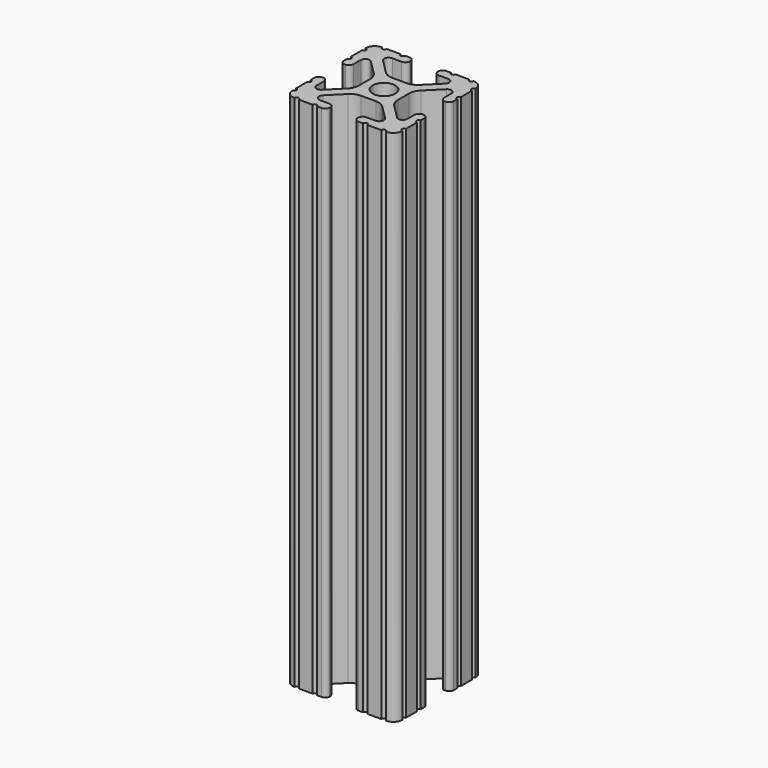
from build123d import *

# Parameters (mm, degrees)
F0_R     = 2.6035
F1_DEPTH = 120


# Not quite as in the source:
# - ends of sketch curves that miss each other by under 0.0002 mm in the source are joined


with BuildPart() as f1:
    # F0 (on Top) → F1 (new body)
    with BuildSketch(Plane.XY):
        with BuildLine():
            ThreePointArc((-3.9522606035, -5.4236922052), (-2.9229262099, -4.7369294977), (-1.7092422, -4.4958))
            Line((-1.7092422, -4.4958), (1.7092422, -4.4958))
            ThreePointArc((1.7092422, -4.4958), (2.9229262099, -4.7369294977), (3.9522606035, -5.4236922052))
            Line((3.9522606035, -5.4236922052), (7.1796402, -8.6451948))
            ThreePointArc((7.1796402, -8.6451948), (7.4147391594, -9.822808991), (6.416421, -10.4902))
            Line((6.416421, -10.4902), (4.28752, -10.4902))
            ThreePointArc((4.28752, -10.4902), (3.5457508444, -10.7974508444), (3.2385, -11.53922))
            Line((3.2385, -11.53922), (3.2385, -11.65098))
            ThreePointArc((3.2385, -11.65098), (3.5457508444, -12.3927491556), (4.28752, -12.7))
            Line((4.28752, -12.7), (5.3171344, -12.7))
            ThreePointArc((5.3171344, -12.7), (5.8251344, -12.192), (6.3331344, -12.7))
            Line((6.3331344, -12.7), (9.5504508, -12.7))
            ThreePointArc((9.5504508, -12.7), (10.0583746, -12.1920000057), (10.5664507771, -12.6998476))
            ThreePointArc((10.5664507771, -12.6998476), (12.0825404752, -12.0825045568), (12.6998469825, -10.5664000074))
            ThreePointArc((12.6998469825, -10.5664000074), (12.1920000057, -10.0583238), (12.7, -9.5504))
            Line((12.7, -9.5504), (12.7, -6.3330836))
            ThreePointArc((12.7, -6.3330836), (12.192, -5.8250836), (12.7, -5.3170836))
            Line((12.7, -5.3170836), (12.7, -4.2874692))
            ThreePointArc((12.7, -4.2874692), (12.3927491556, -3.5457000444), (11.65098, -3.2384492))
            Line((11.65098, -3.2384492), (11.53922, -3.2384492))
            ThreePointArc((11.53922, -3.2384492), (10.7974508444, -3.5457000444), (10.4902, -4.2874692))
            Line((10.4902, -4.2874692), (10.4902, -6.4020954))
            ThreePointArc((10.4902, -6.4020954), (9.8565053438, -7.3510699477), (8.7371366164, -7.1294051977))
            Line((8.7371366164, -7.1294051977), (5.4410102, -3.8408102))
            ThreePointArc((5.4410102, -3.8408102), (4.7508771577, -2.8098852335), (4.5085, -1.5931896))
            Line((4.5085, -1.5931896), (4.5085, 1.5931896))
            ThreePointArc((4.5085, 1.5931896), (4.7508771577, 2.8098852335), (5.4410028439, 3.840817573))
            Line((5.4410028439, 3.840817573), (8.7371428, 7.129399))
            ThreePointArc((8.7371428, 7.129399), (9.8565053438, 7.3510699477), (10.4902, 6.4020954))
            Line((10.4902, 6.4020954), (10.4902, 4.2874692))
            ThreePointArc((10.4902, 4.2874692), (10.7974508444, 3.5457000444), (11.53922, 3.2384492))
            Line((11.53922, 3.2384492), (11.65098, 3.2384492))
            ThreePointArc((11.65098, 3.2384492), (12.3927491556, 3.5457000444), (12.7, 4.2874692))
            Line((12.7, 4.2874692), (12.7, 5.3170836))
            ThreePointArc((12.7, 5.3170836), (12.192, 5.8250836), (12.7, 6.3330836))
            Line((12.7, 6.3330836), (12.7, 9.5504))
            ThreePointArc((12.7, 9.5504), (12.1920000057, 10.0583238), (12.6998476, 10.5663999771))
            ThreePointArc((12.6998476, 10.5663999771), (12.0825404752, 12.0825045568), (10.5664508001, 12.6998475939))
            ThreePointArc((10.5664508001, 12.6998475939), (10.0583746, 12.1920000057), (9.5504508, 12.7))
            Line((9.5504508, 12.7), (6.3331344, 12.7))
            ThreePointArc((6.3331344, 12.7), (5.8251344, 12.192), (5.3171344, 12.7))
            Line((5.3171344, 12.7), (4.28752, 12.7))
            ThreePointArc((4.28752, 12.7), (3.5457508444, 12.3927491556), (3.2385, 11.65098))
            Line((3.2385, 11.65098), (3.2385, 11.53922))
            ThreePointArc((3.2385, 11.53922), (3.5457508444, 10.7974508444), (4.28752, 10.4902))
            Line((4.28752, 10.4902), (6.4767968, 10.4902))
            ThreePointArc((6.4767968, 10.4902), (7.4322289723, 9.8514044384), (7.2070407772, 8.7243726366))
            Line((7.2070407772, 8.7243726366), (3.898265, 5.4231794))
            ThreePointArc((3.898265, 5.4231794), (2.8691189654, 4.7367887684), (1.6557752, 4.4958))
            Line((1.6557752, 4.4958), (-1.6557752, 4.4958))
            ThreePointArc((-1.6557752, 4.4958), (-2.8691189654, 4.7367887684), (-3.8982723561, 5.423172027))
            Line((-3.8982723561, 5.423172027), (-7.2070468, 8.7243666))
            ThreePointArc((-7.2070468, 8.7243666), (-7.4322289723, 9.8514044384), (-6.4767968, 10.4902))
            Line((-6.4767968, 10.4902), (-4.28752, 10.4902))
            ThreePointArc((-4.28752, 10.4902), (-3.5457508444, 10.7974508444), (-3.2385, 11.53922))
            Line((-3.2385, 11.53922), (-3.2385, 11.65098))
            ThreePointArc((-3.2385, 11.65098), (-3.5457508444, 12.3927491556), (-4.28752, 12.7))
            Line((-4.28752, 12.7), (-5.3171344, 12.7))
            ThreePointArc((-5.3171344, 12.7), (-5.8251344, 12.192), (-6.3331344, 12.7))
            Line((-6.3331344, 12.7), (-9.5504508, 12.7))
            ThreePointArc((-9.5504508, 12.7), (-10.0583746, 12.1920000057), (-10.5664507771, 12.6998476))
            ThreePointArc((-10.5664507771, 12.6998476), (-12.0825404752, 12.0825045568), (-12.6998469825, 10.5664000074))
            ThreePointArc((-12.6998469825, 10.5664000074), (-12.1920000057, 10.0583238), (-12.7, 9.5504))
            Line((-12.7, 9.5504), (-12.7, 6.3330836))
            ThreePointArc((-12.7, 6.3330836), (-12.192, 5.8250836), (-12.7, 5.3170836))
            Line((-12.7, 5.3170836), (-12.7, 4.2874692))
            ThreePointArc((-12.7, 4.2874692), (-12.3927491556, 3.5457000444), (-11.65098, 3.2384492))
            Line((-11.65098, 3.2384492), (-11.53922, 3.2384492))
            ThreePointArc((-11.53922, 3.2384492), (-10.7974508444, 3.5457000444), (-10.4902, 4.2874692))
            Line((-10.4902, 4.2874692), (-10.4902, 6.4020954))
            ThreePointArc((-10.4902, 6.4020954), (-9.8565053438, 7.3510699477), (-8.7371366164, 7.1294051977))
            Line((-8.7371366164, 7.1294051977), (-5.4410102, 3.8408102))
            ThreePointArc((-5.4410102, 3.8408102), (-4.7508771577, 2.8098852335), (-4.5085, 1.5931896))
            Line((-4.5085, 1.5931896), (-4.5085, -1.5931896))
            ThreePointArc((-4.5085, -1.5931896), (-4.7508771577, -2.8098852335), (-5.4410028439, -3.840817573))
            Line((-5.4410028439, -3.840817573), (-8.7371428, -7.129399))
            ThreePointArc((-8.7371428, -7.129399), (-9.8565053438, -7.3510699477), (-10.4902, -6.4020954))
            Line((-10.4902, -6.4020954), (-10.4902, -4.2874692))
            ThreePointArc((-10.4902, -4.2874692), (-10.7974508444, -3.5457000444), (-11.53922, -3.2384492))
            Line((-11.53922, -3.2384492), (-11.65098, -3.2384492))
            ThreePointArc((-11.65098, -3.2384492), (-12.3927491556, -3.5457000444), (-12.7, -4.2874692))
            Line((-12.7, -4.2874692), (-12.7, -5.3170836))
            ThreePointArc((-12.7, -5.3170836), (-12.192, -5.8250836), (-12.7, -6.3330836))
            Line((-12.7, -6.3330836), (-12.7, -9.5504))
            ThreePointArc((-12.7, -9.5504), (-12.1920000057, -10.0583238), (-12.6998476, -10.5663999771))
            ThreePointArc((-12.6998476, -10.5663999771), (-12.0825404752, -12.0825045568), (-10.5664508001, -12.6998475939))
            ThreePointArc((-10.5664508001, -12.6998475939), (-10.0583746, -12.1920000057), (-9.5504508, -12.7))
            Line((-9.5504508, -12.7), (-6.3331344, -12.7))
            ThreePointArc((-6.3331344, -12.7), (-5.8251344, -12.192), (-5.3171344, -12.7))
            Line((-5.3171344, -12.7), (-4.28752, -12.7))
            ThreePointArc((-4.28752, -12.7), (-3.5457508444, -12.3927491556), (-3.2385, -11.65098))
            Line((-3.2385, -11.65098), (-3.2385, -11.53922))
            ThreePointArc((-3.2385, -11.53922), (-3.5457508444, -10.7974508444), (-4.28752, -10.4902))
            Line((-4.28752, -10.4902), (-6.416421, -10.4902))
            ThreePointArc((-6.416421, -10.4902), (-7.4147391594, -9.822808991), (-7.1796418951, -8.6451931018))
            Line((-7.1796418951, -8.6451931018), (-3.9522606035, -5.4236922052))
        make_face()
        Circle(F0_R, mode=Mode.SUBTRACT)
    extrude(amount=F1_DEPTH)


solid = f1.part
